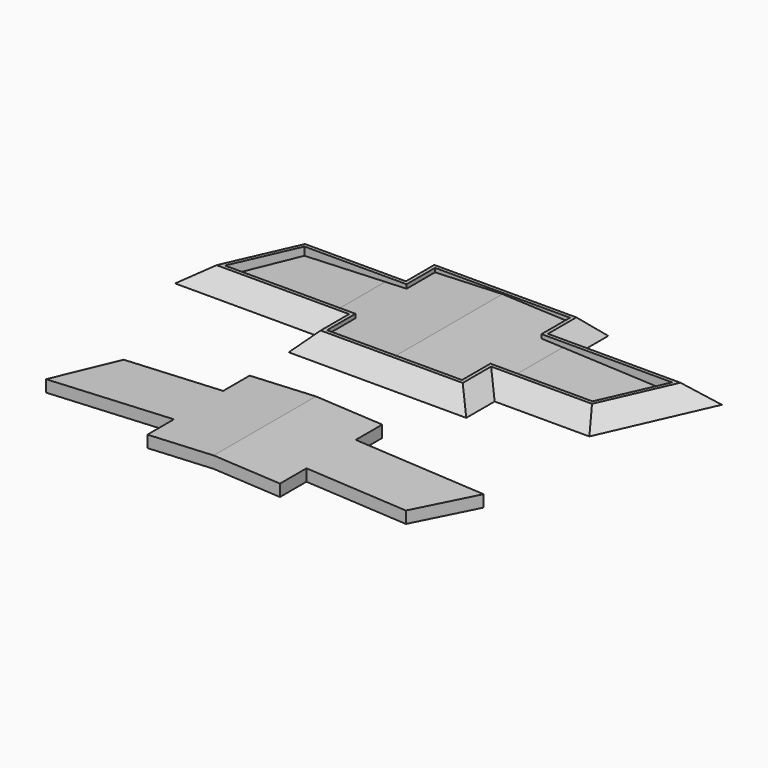
from build123d import *

# Parameters (mm, degrees)
F1_DEPTH  = 9.525
F3_DEPTH  = 6.35
F5_DEPTH  = 83.82
F6_DEPTH  = 3.1271538462
F7_SIZE   = 9.52499
F9_DEPTH  = 6.35
F11_DEPTH = 68.58
F12_DEPTH = 3.3463658537
F14_DEPTH = 68.58
F15_T     = -5.08
F17_DEPTH = 2.54


# Not quite as in the source:
# - a fillet or chamfer is up to 0.001 mm smaller than in the source, because OpenCascade refuses the exact size
# - a length typed as a fraction of an inch, garbled in the dataset ("3 / 203.2 mm" for 3/8 in), is restored


with BuildPart() as f1:
    # F0 (on Top) → F1 (new body)
    with BuildSketch(Plane.XY):
        Polygon((-47.625, 28.575), (-98.425, 28.575), (-123.825, -28.575), (-47.625, -28.575), (-47.625, -47.625), (47.625, -47.625), (47.625, -28.575), (98.425, -28.575), (123.825, 28.575), (47.625, 28.575), (47.625, 47.625), (-47.625, 47.625), align=None)
    extrude(amount=F1_DEPTH)

    # F2 (on face) → F3 (cut)
    with BuildSketch(Plane.XY.offset(9.525)):
        Polygon((-36.195, 36.195), (-36.195, 17.145), (-90.9969505917, 17.145), (-106.2369505917, -17.145), (-36.195, -17.145), (-36.195, -36.195), (36.195, -36.195), (36.195, -17.145), (90.9969505917, -17.145), (106.2369505917, 17.145), (36.195, 17.145), (36.195, 36.195), align=None)
    extrude(amount=-F3_DEPTH, mode=Mode.SUBTRACT)

    # F4 (on face) → F5 (join, through all)
    with BuildSketch(Plane.XZ.offset(47.625)):
        Polygon((-47.625, 6.9361538462), (-47.625, 3.81), (47.625, 3.81), (47.625, 6.9361538462), (0, 8.89), align=None)
        Polygon((-47.625, 6.9361538462), (-123.825, 3.81), (-47.625, 3.81), align=None)
        Polygon((47.625, 6.9361538462), (47.625, 3.81), (123.825, 3.81), align=None)
    extrude(amount=-F5_DEPTH)

    # F6 (cut, through all): faces of the model
    f6_faces = [f1.faces().sort_by_distance(p)[0] for p in [
        (-85.725, -38.1, 3.81),
        (85.725, -46.5473692655, 3.81),
        (85.725, 32.385, 3.81),
        (-112.0388843262, 0.4061708117, 3.81),
    ]]
    extrude(f6_faces, amount=-F6_DEPTH, mode=Mode.SUBTRACT)

    # F7 (size 9.525 in the source; OpenCascade refuses exactly that, so slightly less here)
    f7_edges = [f1.edges().sort_by_distance(p)[0] for p in [
        (-111.125, 0, 9.525),
        (-73.025, 28.575, 9.525),
        (0, 47.625, 9.525),
        (-47.625, 38.1, 9.525),
        (47.625, 38.1, 9.525),
        (85.725, 28.575, 9.525),
        (111.125, 0, 9.525),
        (73.025, -28.575, 9.525),
        (47.625, -38.1, 9.525),
        (0, -47.625, 9.525),
        (-47.625, -38.1, 9.525),
        (-85.725, -28.575, 9.525),
    ]]
    chamfer(f7_edges, length=F7_SIZE)

    # F16 (on face) → F17 (cut)
    with BuildSketch(Plane(origin=(0, 0, 0), x_dir=(1, 0, 0), z_dir=(0, 0, -1))):
        Polygon((-41.275, 41.275), (-41.275, 22.225), (-114.0538614398, 22.225), (-94.2983058843, -22.225), (-41.275, -22.225), (-41.275, -41.275), (41.275, -41.275), (41.275, -22.225), (114.0538614398, -22.225), (94.2983058843, 22.225), (41.275, 22.225), (41.275, 41.275), align=None)
    extrude(amount=-F17_DEPTH, mode=Mode.SUBTRACT)


with BuildPart() as f9:
    # F8 (on Top) → F9 (new body)
    with BuildSketch(Plane.XY):
        Polygon((-35.56, -106.68), (-88.9, -106.68), (-104.14, -139.7), (-35.56, -139.7), (-35.56, -157.48), (35.56, -157.48), (35.56, -139.7), (88.9, -139.7), (104.14, -106.68), (35.56, -106.68), (35.56, -88.9), (-35.56, -88.9), align=None)
    extrude(amount=F9_DEPTH)

    # F10 (on face) → F11 (join, through all)
    with BuildSketch(Plane.XZ.offset(157.48)):
        Polygon((0, 11.43), (-104.14, 6.35), (104.14, 6.35), align=None)
    extrude(amount=-F11_DEPTH)

    # F12 (cut, through all): faces of the model
    f12_faces = [f9.faces().sort_by_distance(p)[0] for p in [
        (-69.85, -148.59, 6.35),
        (-74.8464473684, -101.193377193, 6.35),
        (74.8464473684, -145.186622807, 6.35),
        (69.85, -97.79, 6.35),
    ]]
    extrude(f12_faces, amount=-F12_DEPTH, mode=Mode.SUBTRACT)

    # F13 (on face) → F14 (cut, through all)
    with BuildSketch(Plane.XZ.offset(157.48)):
        Polygon((0, 5.08), (-104.14, 0), (104.14, 0), align=None)
    extrude(amount=-F14_DEPTH, mode=Mode.SUBTRACT)

    # F15
    f15_openings = [f9.faces().sort_by_distance(p)[0] for p in [
        (-39.673696, -123.501058, 3.144698),
        (39.673696, -122.878942, 3.144698),
    ]]
    offset(amount=F15_T, openings=f15_openings, kind=Kind.INTERSECTION)


solid = Compound([f1.part, f9.part])
